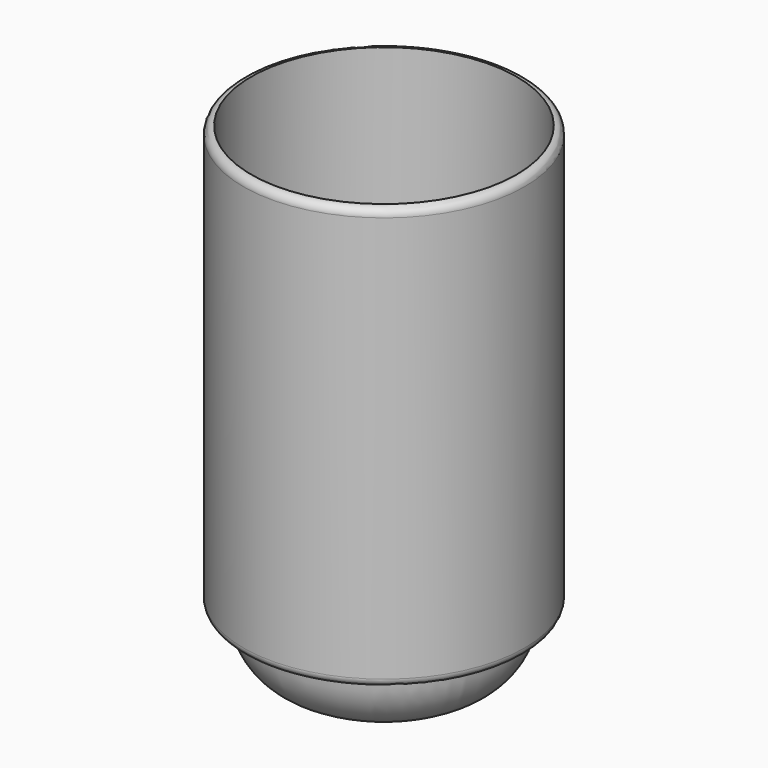
from build123d import *

# Parameters (mm, degrees)
F2_T = -2.54
F3_R = 2.53999
F4_R = 2.54


# Not quite as in the source:
# - a fillet or chamfer is up to 0.001 mm smaller than in the source, because OpenCascade refuses the exact size


with BuildPart() as f1:
    # F0 (on Front) → F1 (revolve)
    with BuildSketch(Plane.XZ):
        with BuildLine():
            Line((0, 152.4), (0, 0))
            Line((0, 0), (25.4, 0))
            ThreePointArc((25.4, 0), (34.9311237351, 7.4042508433), (38.1, 19.05))
            Line((38.1, 19.05), (44.45, 19.05))
            Line((44.45, 19.05), (44.45, 152.4))
            Line((44.45, 152.4), (0, 152.4))
        make_face()
    revolve(axis=Axis((0, 0, 81.1481997371), (0, 0, -1)))

    # F2
    f2_openings = [f1.faces().sort_by_distance(p)[0] for p in [
        (0, 0, 152.4),
    ]]
    offset(amount=F2_T, openings=f2_openings, kind=Kind.INTERSECTION)

    # F3 (radius 2.54 in the source; OpenCascade refuses exactly that, so slightly less here)
    f3_edges = [f1.edges().sort_by_distance(p)[0] for p in [
        (-44.45, 0, 19.05),
        (-44.45, 0, 152.4),
    ]]
    fillet(f3_edges, radius=F3_R)

    # F4
    f4_edges = [f1.edges().sort_by_distance(p)[0] for p in [
        (-25.4, 0, 0),
        (-38.1, 0, 19.05),
        (34.931124, 0, 7.404251),
    ]]
    fillet(f4_edges, radius=F4_R)


solid = f1.part
